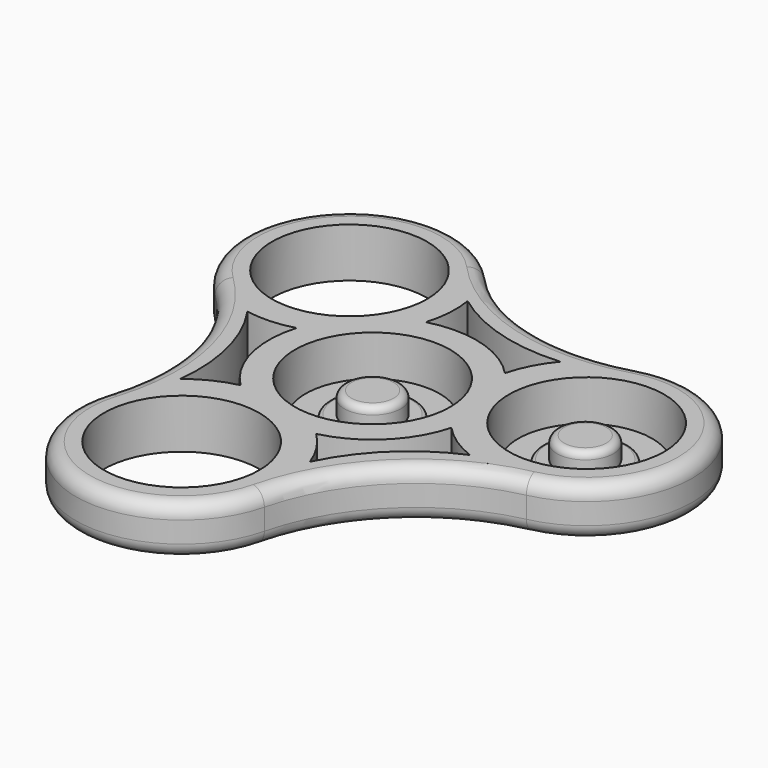
from build123d import *

# Parameters (mm, degrees)
F0_R     = 11
F1_DEPTH = 7
F2_R     = 2
F3_R     = 2
F4_R     = 9.5
F5_DEPTH = 2
F6_R     = 6
F7_DEPTH = 0.5
F8_R     = 4
F9_DEPTH = 3
F10_R    = 1
F11_R    = 0.49999
F12_R    = 1


# Not quite as in the source:
# - a fillet or chamfer is up to 0.001 mm smaller than in the source, because OpenCascade refuses the exact size


with BuildPart() as f1:
    # F0 (on Top) → F1 (new body)
    with BuildSketch(Plane.XY):
        with BuildLine():
            ThreePointArc((-28.5224371489, 7.7688560065), (-20.8782861802, -5.318736508), (-21.328982888, -20.4684887943))
            ThreePointArc((-21.328982888, -20.4684887943), (-11.100071503, -39.4688283666), (7.5331919145, -28.585583152))
            ThreePointArc((7.5331919145, -28.585583152), (15.0453040221, -15.4217579655), (28.390722717, -8.2371966208))
            ThreePointArc((28.390722717, -8.2371966208), (39.7310437745, 10.1214702779), (20.9892452344, 20.8167271455))
            ThreePointArc((20.9892452344, 20.8167271455), (5.8329821581, 20.7404944735), (-7.061739829, 28.7056854151))
            ThreePointArc((-7.061739829, 28.7056854151), (-28.6309722716, 29.3473580887), (-28.5224371489, 7.7688560065))
        make_face()
        with Locations((-7.0390697336, -25.0290131105)):
            Circle(F0_R, mode=Mode.SUBTRACT)
        with BuildLine():
            ThreePointArc((-14.1007848463, 4.1691419046), (-14.2491152943, -3.6299574146), (-10.3873909989, -10.4074966124))
            ThreePointArc((-10.3873909989, -10.4074966124), (-13.6350001052, -11.5570532481), (-16.5346828148, -13.4172375265))
            ThreePointArc((-16.5346828148, -13.4172375265), (-17.1028685976, -4.3943345863), (-20.8168292987, 3.8483657276))
            ThreePointArc((-20.8168292987, 3.8483657276), (-17.4406021548, 3.6276000863), (-14.1007848463, 4.1691419046))
        make_face(mode=Mode.SUBTRACT)
        with BuildLine():
            ThreePointArc((3.4398096218, -14.2962088425), (10.2681929828, -10.525117119), (14.2068519556, -3.7919961779))
            ThreePointArc((14.2068519556, -3.7919961779), (16.8262017584, -6.0297298476), (19.887009954, -7.6108365979))
            ThreePointArc((19.887009954, -7.6108365979), (12.3570396832, -12.61435139), (7.0756321662, -19.9520858627))
            ThreePointArc((7.0756321662, -19.9520858627), (5.5787072479, -16.9178045665), (3.4398096218, -14.2962088425))
        make_face(mode=Mode.SUBTRACT)
        Circle(F0_R, mode=Mode.SUBTRACT)
        with Locations((-18.1562263185, 18.6105197636)):
            Circle(F0_R, mode=Mode.SUBTRACT)
        with Locations((25.1952960521, 6.4184933469)):
            Circle(F0_R, mode=Mode.SUBTRACT)
        with BuildLine():
            ThreePointArc((10.6609752245, 10.1270669379), (3.9809223115, 14.1550745336), (-3.8194609567, 14.1994927903))
            ThreePointArc((-3.8194609567, 14.1994927903), (-3.1912016532, 17.5867830958), (-3.3523271392, 21.0280741244))
            ThreePointArc((-3.3523271392, 21.0280741244), (4.7458289144, 17.0086859762), (13.7411971325, 16.1037201351))
            ThreePointArc((13.7411971325, 16.1037201351), (11.8618949069, 13.2902044802), (10.6609752245, 10.1270669379))
        make_face(mode=Mode.SUBTRACT)
    extrude(amount=F1_DEPTH)

    # F2
    f2_edges = [f1.edges().sort_by_distance(p)[0] for p in [
        (-11.100072, -39.468828, 7),
    ]]
    fillet(f2_edges, radius=F2_R)

    # F3
    f3_edges = [f1.edges().sort_by_distance(p)[0] for p in [
        (15.045304, -15.421758, 0),
    ]]
    fillet(f3_edges, radius=F3_R)


with BuildPart() as f5:
    # F4 (on Top) → F5 (new body)
    with BuildSketch(Plane.XY):
        Circle(F4_R)
    extrude(amount=F5_DEPTH)

    # F6 (on face) → F7 (join)
    with BuildSketch(Plane.XY.offset(2)):
        Circle(F6_R)
    extrude(amount=F7_DEPTH)

    # F8 (on face) → F9 (join)
    with BuildSketch(Plane.XY.offset(2.5)):
        Circle(F8_R)
    extrude(amount=F9_DEPTH)

    # F10
    f10_edges = [f5.edges().sort_by_distance(p)[0] for p in [
        (-4, 0, 5.5),
    ]]
    fillet(f10_edges, radius=F10_R)

    # F11 (radius 0.5 in the source; OpenCascade refuses exactly that, so slightly less here)
    f11_edges = [f5.edges().sort_by_distance(p)[0] for p in [
        (-6, 0, 2.5),
    ]]
    fillet(f11_edges, radius=F11_R)

    # F12
    f12_edges = [f5.edges().sort_by_distance(p)[0] for p in [
        (-9.5, 0, 0),
    ]]
    fillet(f12_edges, radius=F12_R)


with BuildPart() as f13_1:
    # F13: copy of F5
    add(f5.part.moved(Location((25.1, 6.3, 0))))


solid = Compound([f1.part, f5.part, f13_1.part])
